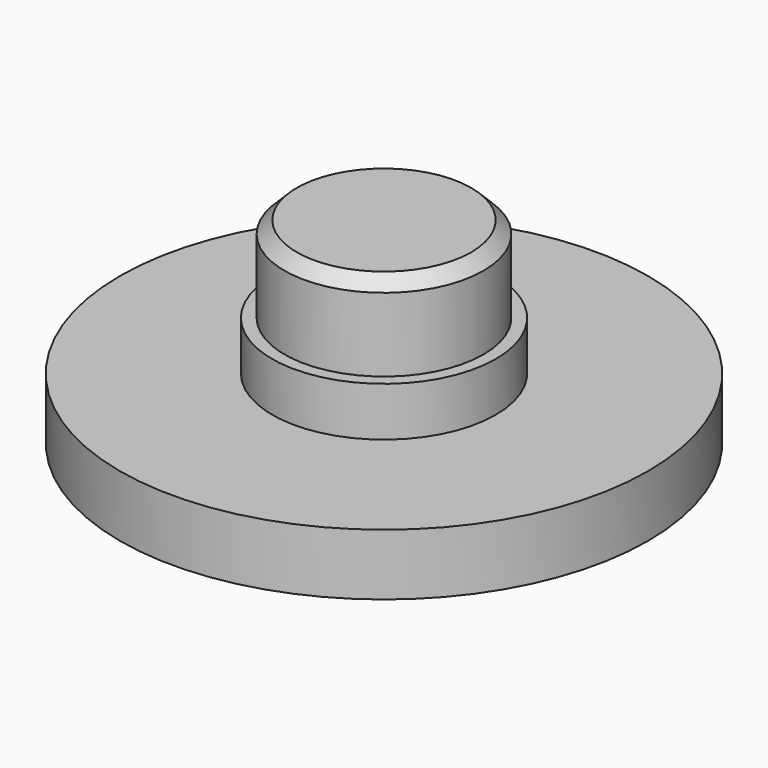
from build123d import *

# Parameters (mm, degrees)
F0_R     = 10.75
F1_DEPTH = 2.5
F2_R     = 4.05
F3_DEPTH = 5.5
F4_SIZE  = 0.5
F5_R     = 4.55
F6_DEPTH = 2
F7_DEPTH = 0.5


# Not quite as in the source:
# - a feature names something its author has since deleted; it is built from what else it names


with BuildPart() as f1:
    # F0 (on Top) → F1 (new body)
    with BuildSketch(Plane.XY):
        Circle(F0_R)
        with BuildLine():
            ThreePointArc((0, -10), (-7.0710678119, 7.0710678119), (10, 0))
            ThreePointArc((10, 0), (7.0710678119, -7.0710678119), (0, -10))
        make_face(mode=Mode.SUBTRACT)
        with BuildLine():
            ThreePointArc((0, -10), (7.0710678119, -7.0710678119), (10, 0))
            ThreePointArc((10, 0), (-7.0710678119, 7.0710678119), (0, -10))
        make_face()
        Polygon((3.1044567973, -4.3237269842), (0, -10), (-3.1044567973, -4.3237269842), (-9.4622431459, -3.1252779442), (-5.0231166146, 1.581300749), (-5.847987874, 7.9982560054), (0, 5.2308085927), (5.847987874, 7.9982560054), (5.0231166146, 1.581300749), (9.4622431459, -3.1252779442), align=None, mode=Mode.SUBTRACT)
        Polygon((-3.1044567973, -4.3237269842), (0, -10), (3.1044567973, -4.3237269842), (9.4622431459, -3.1252779442), (5.0231166146, 1.581300749), (5.847987874, 7.9982560054), (0, 5.2308085927), (-5.847987874, 7.9982560054), (-5.0231166146, 1.581300749), (-9.4622431459, -3.1252779442), align=None)
    extrude(amount=F1_DEPTH)

    # F2 (on face) → F3 (join)
    with BuildSketch(Plane.XY.offset(2.5)):
        Circle(F2_R)
    extrude(amount=F3_DEPTH)

    # F4
    f4_edges = [f1.edges().sort_by_distance(p)[0] for p in [
        (-4.05, 0, 8),
    ]]
    chamfer(f4_edges, length=F4_SIZE)

    # F5 (on face) → F6 (join)
    with BuildSketch(Plane.XY.offset(2.5)):
        Circle(F5_R)
    extrude(amount=F6_DEPTH)

    # F0 (on Top) → F7 (cut)
    with BuildSketch(Plane.XY):
        Polygon((-3.1044567973, -4.3237269842), (0, -10), (3.1044567973, -4.3237269842), (9.4622431459, -3.1252779442), (5.0231166146, 1.581300749), (5.847987874, 7.9982560054), (0, 5.2308085927), (-5.847987874, 7.9982560054), (-5.0231166146, 1.581300749), (-9.4622431459, -3.1252779442), align=None)
    extrude(amount=F7_DEPTH, mode=Mode.SUBTRACT)


solid = f1.part
